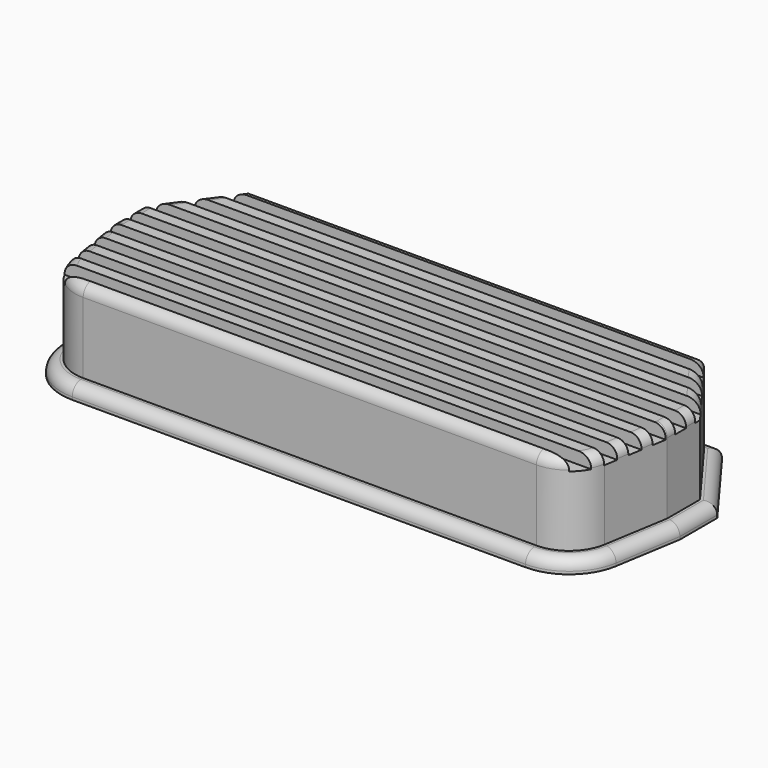
from build123d import *

# Parameters (mm, degrees)
F1_DEPTH     = 44.45
F2_DEPTH     = 6.35
F3_R         = 5.08
F4_W         = 6.35
F4_H         = 12.7
F5_DEPTH     = 381
F6_T         = 1.27
F6_T3_DEPTH  = 21.6242188895
F6_T5_DEPTH  = 260.9417800188
F6_T7_DEPTH  = 255.6296420558
F6_T9_DEPTH  = 42.2029136982
F6_T11_DEPTH = 213.3671407514
F6_T13_DEPTH = 33.2308036091
F6_T15_DEPTH = 213.7688177013
F6_T17_DEPTH = 42.2029136982
F6_T19_DEPTH = 33.2308036091
F6_T21_DEPTH = 247.738803967
F6_T23_DEPTH = 238.3449490995
F6_T25_DEPTH = 230.4541110108
F6_T27_DEPTH = 221.0602561433
F6_T29_DEPTH = 250.9166851773
F6_T31_DEPTH = 253.0107074871
F6_T33_DEPTH = 254.7689257871
F6_T35_DEPTH = 256.8620428108
F6_T37_DEPTH = 258.6202611107
F6_T39_DEPTH = 260.7133781345
F6_T41_DEPTH = 247.4035921048
F6_T43_DEPTH = 237.0803359817
F6_T46_ANGLE = 80.6410810347
F6_T48_ANGLE = 80.6410810347


# Not quite as in the source:
# - a shell that OpenCascade refuses in one call is made with other operations: the cavity is built on its own and cut out


with BuildPart() as f1:
    # F0 (on Top) → F1 (new body)
    with BuildSketch(Plane.XY):
        with BuildLine():
            ThreePointArc((-221.9209556791, -63.7008499126), (-215.4510830778, -75.1273801076), (-203.124529989, -79.6529665584))
            Line((-203.124529989, -79.6529665584), (7.7026107624, -79.6529665584))
            ThreePointArc((7.7026107624, -79.6529665584), (20.0291638512, -75.1273801076), (26.4990364525, -63.7008499126))
            Line((26.4990364525, -63.7008499126), (31.4899303961, -33.4185712034))
            Line((31.4899303961, -33.4185712034), (31.4899303961, -14.334352314))
            Line((31.4899303961, -14.334352314), (7.9034492373, 17.5533354287))
            Line((7.9034492373, 17.5533354287), (-203.325368464, 17.5533354287))
            Line((-203.325368464, 17.5533354287), (-226.9118496227, -14.334352314))
            Line((-226.9118496227, -14.334352314), (-226.9118496227, -33.4185712034))
            Line((-226.9118496227, -33.4185712034), (-221.9209556791, -63.7008499126))
        make_face()
    extrude(amount=F1_DEPTH)

    # F0 (on Top) → F2 (join)
    with BuildSketch(Plane.XY):
        with BuildLine():
            Line((-233.2618496227, -33.9383444433), (-228.1864309092, -64.7334776973))
            ThreePointArc((-228.1864309092, -64.7334776973), (-219.5599341074, -79.9688512907), (-203.124529989, -86.0029665584))
            Line((-203.124529989, -86.0029665584), (7.7026107624, -86.0029665584))
            ThreePointArc((7.7026107624, -86.0029665584), (24.1380148808, -79.9688512907), (32.7645116825, -64.7334776973))
            Line((32.7645116825, -64.7334776973), (37.8399303961, -33.9383444433))
            Line((37.8399303961, -33.9383444433), (37.8399303961, -12.24109031))
            Line((37.8399303961, -12.24109031), (11.1048524701, 23.9033354287))
            Line((11.1048524701, 23.9033354287), (-206.5267716968, 23.9033354287))
            Line((-206.5267716968, 23.9033354287), (-233.2618496227, -12.24109031))
            Line((-233.2618496227, -12.24109031), (-233.2618496227, -33.9383444433))
        make_face()
        with BuildLine():
            Line((7.7026107624, -79.6529665584), (-203.124529989, -79.6529665584))
            ThreePointArc((-203.124529989, -79.6529665584), (-215.4510830778, -75.1273801076), (-221.9209556791, -63.7008499126))
            Line((-221.9209556791, -63.7008499126), (-226.9118496227, -33.4185712034))
            Line((-226.9118496227, -33.4185712034), (-226.9118496227, -14.334352314))
            Line((-226.9118496227, -14.334352314), (-203.325368464, 17.5533354287))
            Line((-203.325368464, 17.5533354287), (7.9034492373, 17.5533354287))
            Line((7.9034492373, 17.5533354287), (31.4899303961, -14.334352314))
            Line((31.4899303961, -14.334352314), (31.4899303961, -33.4185712034))
            Line((31.4899303961, -33.4185712034), (26.4990364525, -63.7008499126))
            ThreePointArc((26.4990364525, -63.7008499126), (20.0291638512, -75.1273801076), (7.7026107624, -79.6529665584))
        make_face(mode=Mode.SUBTRACT)
    extrude(amount=F2_DEPTH)

    # F3
    f3_edges = [f1.edges().sort_by_distance(p)[0] for p in [
        (-226.91185, -23.876462, 44.45),
        (-224.416403, -48.559711, 44.45),
        (-215.451083, -75.12738, 44.45),
        (-97.71096, -79.652967, 44.45),
        (20.029164, -75.12738, 44.45),
        (28.994483, -48.559711, 44.45),
        (31.48993, -23.876462, 44.45),
        (19.69669, 1.609492, 44.45),
        (-97.71096, 17.553335, 44.45),
        (-215.118609, 1.609492, 44.45),
        (-219.894311, 5.831123, 6.35),
        (-233.26185, -23.089717, 6.35),
        (-230.72414, -49.335911, 6.35),
        (-97.71096, 23.903335, 6.35),
        (37.83993, -23.089717, 6.35),
        (24.472391, 5.831123, 6.35),
        (-219.559934, -79.968851, 6.35),
        (-97.71096, -86.002967, 6.35),
        (24.138015, -79.968851, 6.35),
        (35.302221, -49.335911, 6.35),
    ]]
    fillet(f3_edges, radius=F3_R)

    # F4 (on Right) → F5 (cut, symmetric)
    with BuildSketch(Plane.YZ):
        with Locations((9.4495139003, 45.2093561947)):
            Rectangle(F4_W, F4_H)
        with Locations((-2.2344860997, 45.2093561947)):
            Rectangle(F4_W, F4_H)
        with Locations((-13.9184860997, 45.2093561947)):
            Rectangle(F4_W, F4_H)
        with Locations((-25.6024860997, 45.2093561947)):
            Rectangle(F4_W, F4_H)
        with Locations((-37.2864860997, 45.2093561947)):
            Rectangle(F4_W, F4_H)
        with Locations((-48.9704860997, 45.2093561947)):
            Rectangle(F4_W, F4_H)
        with Locations((-60.6544860997, 45.2093561947)):
            Rectangle(F4_W, F4_H)
        with Locations((-72.3384860997, 45.2093561947)):
            Rectangle(F4_W, F4_H)
    extrude(amount=F5_DEPTH, both=True, mode=Mode.SUBTRACT)

    # F6: shell of thickness 1.27, made by hand


with BuildPart() as f6_core1:
    # F6_t2: copy of F1
    add(f1.part)

    # the walls: a layer under each face that stays
    f6_faces = [f6_core1.faces().sort_by_distance(p)[0] for p in [
        (-226.9118496227, -23.8764617587, 22.86),
        (-225.4239516837, -31.0980286516, 42.9621028359),
        (-97.7109596133, -28.7774860997, 41.6546780974),
        (-97.7109596133, -25.6024860997, 38.8593561947),
        (-97.7109596133, -22.4274860997, 41.6546780974),
        (-225.4239520712, -19.7604860997, 42.9621024484),
        (-97.7109596133, -17.0934860997, 41.6546780974),
        (-97.7109596133, -13.9184860997, 38.8593561947),
        (-215.1186090434, 1.6094915574, 22.86),
        (-219.4837902888, -70.9483363597, 6.35),
        (-224.4164026509, -48.559710558, 22.86),
        (-225.3185806728, -33.9361199619, 42.9621028359),
        (-97.7109596133, -31.4444860997, 44.45),
        (30.0020327557, -31.0980286516, 42.9621025373),
        (31.4899303961, -23.8764617587, 22.86),
        (30.0020328445, -19.7604860997, 42.9621024484),
        (-97.7109596133, -19.7604860997, 44.45),
        (19.6966898167, 1.6094915574, 22.86),
        (-97.7109596133, -10.7434860997, 41.6546780974),
        (-219.9695948731, -7.450828722, 42.9621024484),
        (-97.7109596133, -5.4094860997, 41.6546780974),
        (-97.7109596133, -2.2344860997, 38.8593561947),
        (-97.7109596133, 0.9405139003, 41.6546780974),
        (-211.327248395, 4.233171278, 42.9621024484),
        (-97.7109596133, 6.2745139003, 41.6546780974),
        (-97.7109596133, 9.4495139003, 38.8593561947),
        (-97.7109596133, 12.6245139003, 41.6535530977),
        (-203.9946637662, 14.2356635864, 42.9082490984),
        (-97.7109596133, 17.5533354287, 22.86),
        (-218.6980896035, 4.9463094104, 4.8621024484),
        (-97.7109596133, 22.4154378772, 4.8621024484),
        (-231.7739517904, -23.0897173767, 4.8621027292),
        (23.2761703769, 4.9463094104, 4.8621024484),
        (-229.2560478229, -49.0939512841, 4.8621027292),
        (36.3520328445, -23.0897173767, 4.8621024484),
        (-218.5971704245, -78.8344240278, 4.8621024484),
        (33.8341288733, -49.0939513297, 4.8621024484),
        (-97.7109596133, -84.5150690069, 4.8621024484),
        (23.1752511979, -78.8344240278, 4.8621024484),
        (20.0291638512, -75.1273801076, 22.86),
        (-97.7109596133, -79.6529665584, 22.86),
        (-215.4510830778, -75.1273801076, 22.86),
        (28.9944834243, -48.559710558, 22.86),
        (-97.7109596133, -60.6544860997, 38.8593561947),
        (-97.7109596133, -57.4794860997, 41.6546780974),
        (-221.8496998353, -54.983577473, 42.9621024484),
        (-97.7109596133, -52.1454860997, 41.6546780974),
        (-97.7109596133, -48.9704860997, 38.8593561947),
        (-97.7109596133, -45.7954860997, 41.6546780974),
        (-223.7753674971, -43.299577473, 42.9621024484),
        (-97.7109596133, -40.4614860997, 41.6546780974),
        (-97.7109596133, -37.2864860997, 38.8593561947),
        (-97.7109596133, -34.1114860997, 41.6546780974),
        (29.8966617408, -33.9361200105, 42.9621025373),
        (8.5727445392, 14.2356635861, 42.9082490988),
        (15.9053291683, 4.233171278, 42.9621024484),
        (24.5476756464, -7.450828722, 42.9621024484),
        (-97.7109596133, -8.0764860997, 44.45),
        (-97.7109596133, 3.6075139003, 44.45),
        (-97.7109596133, 16.1184956879, 42.9082490988),
        (-219.8943106597, 5.8311225594, 0.635),
        (-97.7109596133, 23.9033354287, 0.635),
        (-233.2618496227, -23.0897173767, 0.635),
        (24.4723914331, 5.8311225594, 0.635),
        (-230.7241402659, -49.3359110703, 0.635),
        (37.8399303961, -23.0897173767, 0.635),
        (-219.5599341074, -79.9688512907, 0.635),
        (35.3022210393, -49.3359110703, 0.635),
        (-97.7109596133, -86.0029665584, 0.635),
        (24.1380148808, -79.9688512907, 0.635),
        (-97.7109596133, -63.8294860997, 41.6546780974),
        (23.7748140195, -67.6819301034, 42.9621024484),
        (-97.7109596133, -69.1634860997, 41.6546780974),
        (-97.7109596133, -72.3384860997, 38.8593561947),
        (-97.7109596133, -75.5134860997, 41.6107661864),
        (13.5963433802, -77.4842193625, 42.6125731087),
        (-97.7109599133, -78.4834805444, 42.6125731087),
        (-209.0182626068, -77.4842193625, 42.6125731087),
        (-219.1967332461, -67.6819301034, 42.9621024484),
        (28.3534482705, -43.299577473, 42.9621024484),
        (26.4277806086, -54.983577473, 42.9621024484),
        (-97.7109596133, -54.8124860997, 44.45),
        (-97.7109596133, -43.1284860997, 44.45),
        (-97.7109596133, -66.4964860997, 44.45),
    ]]
    thicken(f6_faces, amount=-F6_T, mode=Mode.SUBTRACT)

    # F6_s4 → F6_t3 (cut)
    with BuildSketch(Plane.XZ.offset(13.064352314)):
        Polygon((-226.9245496227, 6.3627), (-225.6418496227, 6.35), (-225.6418496227, 5.08), (-226.9118496227, 5.08), align=None)
        Polygon((31.5026303961, 6.3627), (31.4899303961, 5.08), (30.2199303961, 5.08), (30.2199303961, 6.35), align=None)
    extrude(amount=F6_T3_DEPTH, mode=Mode.SUBTRACT)

    # F6_s6 → F6_t5 (cut)
    with BuildSketch(Plane.YZ.offset(-228.1818496227)):
        Polygon((-28.7647860997, 38.8720561947), (-30.0474860997, 38.8593561947), (-30.0474860997, 37.5893561947), (-28.7774860997, 37.5893561947), align=None)
        Polygon((-22.4401860997, 38.8720561947), (-22.4274860997, 37.5893561947), (-21.1574860997, 37.5893561947), (-21.1574860997, 38.8593561947), align=None)
        Polygon((-17.0807860997, 38.8720561947), (-18.3634860997, 38.8593561947), (-18.3634860997, 37.5893561947), (-17.0934860997, 37.5893561947), align=None)
    extrude(amount=F6_T5_DEPTH, mode=Mode.SUBTRACT)

    # F6_s8 → F6_t7 (cut)
    with BuildSketch(Plane.YZ.offset(-225.5257806412)):
        Polygon((-10.7561860997, 38.8720561947), (-10.7434860997, 37.5893561947), (-9.4734860997, 37.5893561947), (-9.4734860997, 38.8593561947), align=None)
    extrude(amount=F6_T7_DEPTH, mode=Mode.SUBTRACT)

    # F6_s10 → F6_t9 (cut)
    with BuildSketch(Plane(origin=(-87.8527720415, -118.7723485898, 0), x_dir=(0, 0, 1), z_dir=(0.5946734357, 0.8039673531, 0))):
        Polygon((6.3627, -173.9181605924), (6.35, -172.6354605924), (5.08, -172.6354605924), (5.08, -173.9054605924), align=None)
    extrude(amount=F6_T9_DEPTH, mode=Mode.SUBTRACT)

    # F6_s12 → F6_t11 (cut)
    with BuildSketch(Plane.YZ.offset(-204.394529989)):
        Polygon((-79.6656665584, 6.3627), (-79.6529665584, 5.08), (-78.3829665584, 5.08), (-78.3829665584, 6.35), align=None)
    extrude(amount=F6_T11_DEPTH, mode=Mode.SUBTRACT)

    # F6_s14 → F6_t13 (cut)
    with BuildSketch(Plane(origin=(4.5589240054, -27.6612985378, 0), x_dir=(0, 0, 1), z_dir=(-0.1626185488, 0.9866890126, 0))):
        Polygon((6.3627, -229.3386084037), (5.08, -229.3259084037), (5.08, -228.0559084037), (6.35, -228.0559084037), align=None)
    extrude(amount=F6_T13_DEPTH, mode=Mode.SUBTRACT)

    # F6_s16 → F6_t15 (cut)
    with BuildSketch(Plane.YZ.offset(-204.595368464)):
        Polygon((17.5660354287, 6.3627), (17.5533354287, 5.08), (16.2833354287, 5.08), (16.2833354287, 6.35), align=None)
    extrude(amount=F6_T15_DEPTH, mode=Mode.SUBTRACT)

    # F6_s18 → F6_t17 (cut)
    with BuildSketch(Plane(origin=(-6.3525022301, 8.5882504531, 0), x_dir=(0, 0, 1), z_dir=(0.5946734357, -0.8039673531, 0))):
        Polygon((6.3627, -16.8053174512), (5.08, -16.7926174512), (5.08, -15.5226174512), (6.35, -15.5226174512), align=None)
    extrude(amount=F6_T17_DEPTH, mode=Mode.SUBTRACT)

    # F6_s20 → F6_t19 (cut)
    with BuildSketch(Plane(origin=(-4.3228710333, -26.2290457245, 0), x_dir=(0, 0, 1), z_dir=(-0.1626185488, -0.9866890126, 0))):
        Polygon((6.3627, -36.5179478807), (5.08, -36.5052478807), (5.08, -35.2352478807), (6.35, -35.2352478807), align=None)
    extrude(amount=F6_T19_DEPTH, mode=Mode.SUBTRACT)

    # F6_s22 → F6_t21 (cut)
    with BuildSketch(Plane.YZ.offset(-221.5803615968)):
        Polygon((-5.3967860997, 38.8720561947), (-6.6794860997, 38.8593561947), (-6.6794860997, 37.5893561947), (-5.4094860997, 37.5893561947), align=None)
    extrude(amount=F6_T21_DEPTH, mode=Mode.SUBTRACT)

    # F6_s24 → F6_t23 (cut)
    with BuildSketch(Plane.YZ.offset(-216.8834341631)):
        Polygon((0.9278139003, 38.8720561947), (0.9405139003, 37.5893561947), (2.2105139003, 37.5893561947), (2.2105139003, 38.8593561947), align=None)
    extrude(amount=F6_T23_DEPTH, mode=Mode.SUBTRACT)

    # F6_s26 → F6_t25 (cut)
    with BuildSketch(Plane.YZ.offset(-212.9380151187)):
        Polygon((6.2872139003, 38.8720561947), (5.0045139003, 38.8593561947), (5.0045139003, 37.5893561947), (6.2745139003, 37.5893561947), align=None)
    extrude(amount=F6_T25_DEPTH, mode=Mode.SUBTRACT)

    # F6_s28 → F6_t27 (cut)
    with BuildSketch(Plane.YZ.offset(-208.241087685)):
        Polygon((12.6118139003, 38.8720561947), (12.6245139003, 37.5893561947), (13.8945139003, 37.5893561947), (13.8945139003, 38.8593561947), align=None)
    extrude(amount=F6_T27_DEPTH, mode=Mode.SUBTRACT)

    # F6_s30 → F6_t29 (cut)
    with BuildSketch(Plane.YZ.offset(-223.169302202)):
        Polygon((-63.8167860997, 38.8720561947), (-63.8294860997, 37.5893561947), (-65.0994860997, 37.5893561947), (-65.0994860997, 38.8593561947), align=None)
    extrude(amount=F6_T29_DEPTH, mode=Mode.SUBTRACT)

    # F6_s32 → F6_t31 (cut)
    with BuildSketch(Plane.YZ.offset(-224.2163133569)):
        Polygon((-57.4921860997, 38.8720561947), (-57.4794860997, 37.5893561947), (-56.2094860997, 37.5893561947), (-56.2094860997, 38.8593561947), align=None)
    extrude(amount=F6_T31_DEPTH, mode=Mode.SUBTRACT)

    # F6_s34 → F6_t33 (cut)
    with BuildSketch(Plane.YZ.offset(-225.0954225069)):
        Polygon((-52.1327860997, 38.8720561947), (-53.4154860997, 38.8593561947), (-53.4154860997, 37.5893561947), (-52.1454860997, 37.5893561947), align=None)
    extrude(amount=F6_T33_DEPTH, mode=Mode.SUBTRACT)

    # F6_s36 → F6_t35 (cut)
    with BuildSketch(Plane.YZ.offset(-226.1419810187)):
        Polygon((-45.8081860997, 38.8720561947), (-45.7954860997, 37.5893561947), (-44.5254860997, 37.5893561947), (-44.5254860997, 38.8593561947), align=None)
    extrude(amount=F6_T35_DEPTH, mode=Mode.SUBTRACT)

    # F6_s38 → F6_t37 (cut)
    with BuildSketch(Plane.YZ.offset(-227.0210901687)):
        Polygon((-40.4487860997, 38.8720561947), (-41.7314860997, 38.8593561947), (-41.7314860997, 37.5893561947), (-40.4614860997, 37.5893561947), align=None)
    extrude(amount=F6_T37_DEPTH, mode=Mode.SUBTRACT)

    # F6_s40 → F6_t39 (cut)
    with BuildSketch(Plane.YZ.offset(-228.0676486806)):
        Polygon((-34.1241860997, 38.8720561947), (-34.1114860997, 37.5893561947), (-32.8414860997, 37.5893561947), (-32.8414860997, 38.8593561947), align=None)
    extrude(amount=F6_T39_DEPTH, mode=Mode.SUBTRACT)

    # F6_s42 → F6_t41 (cut)
    with BuildSketch(Plane.YZ.offset(-221.4127556657)):
        Polygon((-69.1761860997, 38.8720561947), (-67.8934860997, 38.8593561947), (-67.8934860997, 37.5893561947), (-69.1634860997, 37.5893561947), align=None)
    extrude(amount=F6_T41_DEPTH, mode=Mode.SUBTRACT)

    # F6_s44 → F6_t43 (cut)
    with BuildSketch(Plane.YZ.offset(-216.2511276042)):
        Polygon((-75.5007860997, 38.8720561947), (-75.5134860997, 37.5893561947), (-76.7834860997, 37.5893561947), (-76.7834860997, 38.8593561947), align=None)
    extrude(amount=F6_T43_DEPTH, mode=Mode.SUBTRACT)

    # F6_s45 → F6_t46 (revolve, cut)
    with BuildSketch(Plane(origin=(-9.5202905338, -57.7644194796, 0), x_dir=(0, 0, 1), z_dir=(0.1626185488, 0.9866890126, 0))):
        Polygon((6.3627, 36.5179478807), (5.08, 36.5052478807), (5.08, 35.2352478807), (6.35, 35.2352478807), align=None)
    revolve(axis=Axis((7.7026107624, -60.6029665584, 6.35), (0, 0, -1)), revolution_arc=F6_T46_ANGLE, mode=Mode.SUBTRACT)

    # F6_s47 → F6_t48 (revolve, cut)
    with BuildSketch(Plane.YZ.offset(-203.124529989)):
        Polygon((-79.6656665584, 6.3627), (-79.6529665584, 5.08), (-78.3829665584, 5.08), (-78.3829665584, 6.35), align=None)
    revolve(axis=Axis((-203.124529989, -60.6029665584, 6.35), (0, 0, -1)), revolution_arc=F6_T48_ANGLE, mode=Mode.SUBTRACT)


with BuildPart() as f1_1:
    add(f1.part)

    # what is left inside the walls is the cavity
    f6_cavity = [f6_core1.part.solids().sort_by_distance(p)[0] for p in [
        (-97.71096, -48.944199, 0.0127),
    ]]
    add(f6_cavity, mode=Mode.SUBTRACT)


solid = f1_1.part
